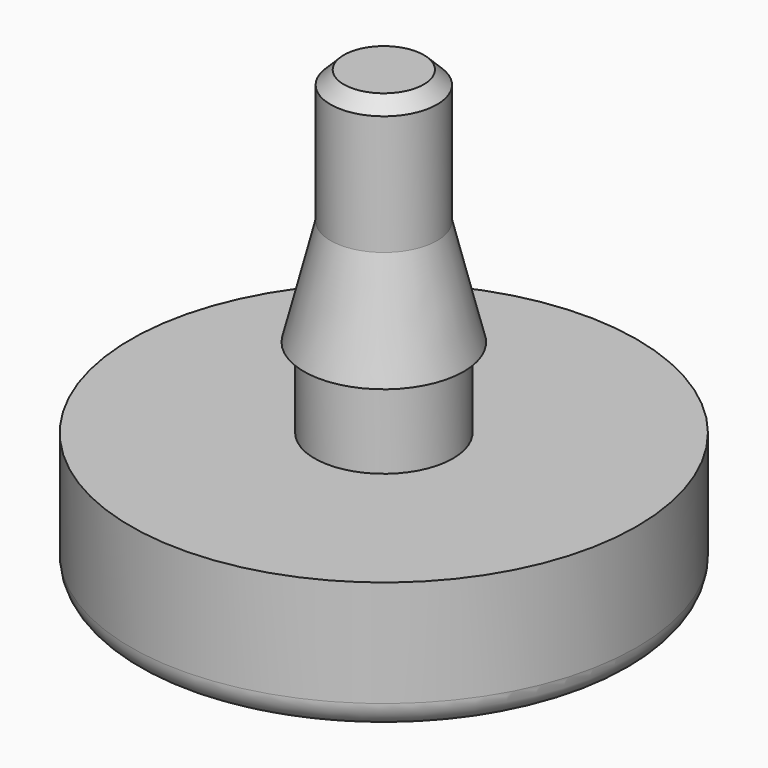
from build123d import *

# Parameters (mm, degrees)
F0_R      = 9.5
F1_DEPTH  = 5
F2_R      = 1
F4_R      = 3
F6_R      = 2
F8_R      = 2.6
F9_DEPTH  = 3
F10_DEPTH = 5
F11_SIZE  = 0.5


with BuildPart() as f1:
    # F0 (on Top) → F1 (new body)
    with BuildSketch(Plane.XY):
        Circle(F0_R)
    extrude(amount=F1_DEPTH)

    # F2
    f2_edges = [f1.edges().sort_by_distance(p)[0] for p in [
        (-9.5, 0, 0),
    ]]
    fillet(f2_edges, radius=F2_R)



with BuildPart() as f7:
    # F4 (on offset) → F7 section 0
    with BuildSketch(Plane.XY.offset(8)):
        Circle(F4_R)
    # F6 (on offset) → F7 section 1
    with BuildSketch(Plane.XY.offset(12)):
        Circle(F6_R)
    loft()


with BuildPart() as f1_1:
    add(f1.part)

    add(f7.part)  # F9 merges F7
    # F8 (on face) → F9 (join)
    with BuildSketch(Plane.XY.offset(5)):
        Circle(F8_R)
    extrude(amount=F9_DEPTH)

    # F10 (add): a face of the model
    f10_faces = [f1_1.faces().sort_by_distance(p)[0] for p in [
        (0, 0, 12),
    ]]
    extrude(f10_faces, amount=F10_DEPTH)

    # F11
    f11_edges = [f1_1.edges().sort_by_distance(p)[0] for p in [
        (-2, 0, 17),
    ]]
    chamfer(f11_edges, length=F11_SIZE)


solid = f1_1.part
